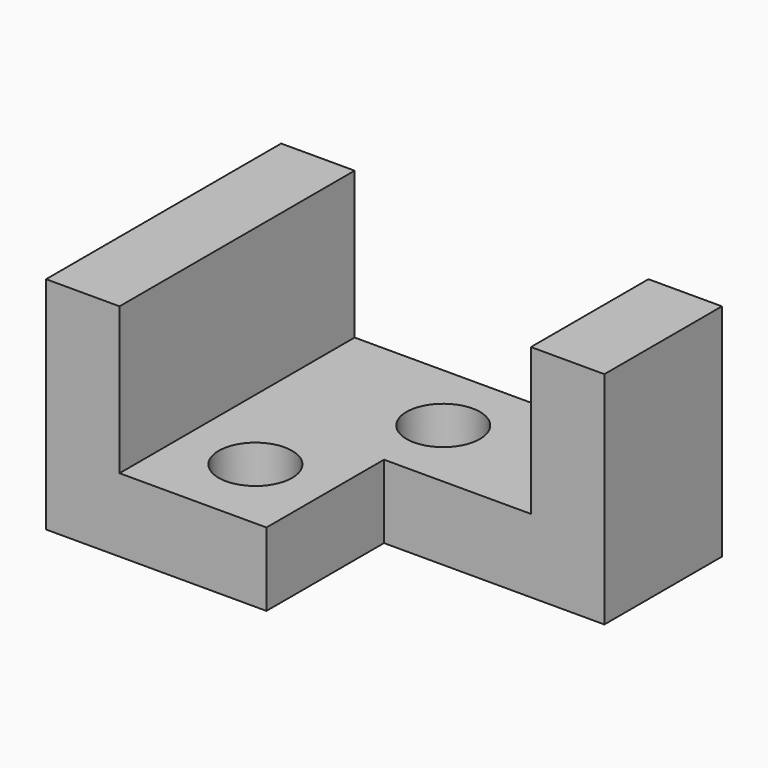
from build123d import *

# Parameters (mm, degrees)
F0_W      = 76.2
F0_H      = 12.7
F1_DEPTH  = 25.4
F3_DEPTH  = 50.8
F4_W      = 38.1
F4_H      = 12.7
F5_DEPTH  = 25.4
F6_W      = 12.7
F6_H      = 25.4
F7_DEPTH  = 25.4
F8_W      = 12.7
F8_H      = 50.8
F9_DEPTH  = 25.4
F10_R     = 6.35
F11_DEPTH = 25.4
F12_R     = 6.35
F13_DEPTH = 25.4


# Not quite as in the source:
# - a feature of the source that left no trace in its solid (it failed there, or was rolled back) is left out


with BuildPart() as f1:
    # F0 (on Front) → F1 (new body)
    with BuildSketch(Plane.XZ):
        with Locations((4.0105291711, 0)):
            Rectangle(F0_W, F0_H)
    extrude(amount=F1_DEPTH)

    # F0 (on Front) → F3 (join)
    with BuildSketch(Plane.XZ):
        with Locations((4.0105291711, 0)):
            Rectangle(F0_W, F0_H)
    extrude(amount=F3_DEPTH)

    # F4 (on face) → F5 (cut)
    with BuildSketch(Plane.XZ.offset(50.8)):
        with Locations((23.0605291711, 0)):
            Rectangle(F4_W, F4_H)
    extrude(amount=-F5_DEPTH, mode=Mode.SUBTRACT)

    # F6 (on face) → F7 (join)
    with BuildSketch(Plane.XY.offset(6.35)):
        with Locations((35.7605291711, -12.7)):
            Rectangle(F6_W, F6_H)
    extrude(amount=F7_DEPTH)

    # F8 (on face) → F9 (join)
    with BuildSketch(Plane.XY.offset(6.35)):
        with Locations((-27.7394708289, -25.4)):
            Rectangle(F8_W, F8_H)
    extrude(amount=F9_DEPTH)

    # F10 (on face) → F11 (cut)
    with BuildSketch(Plane.XY.offset(6.35)):
        with Locations((-8.6894708289, -37.3077057302)):
            Circle(F10_R)
    extrude(amount=-F11_DEPTH, mode=Mode.SUBTRACT)

    # F12 (on face) → F13 (cut)
    with BuildSketch(Plane.XY.offset(6.35)):
        with Locations((4.0105291711, -12.5951375812)):
            Circle(F12_R)
    extrude(amount=-F13_DEPTH, mode=Mode.SUBTRACT)


solid = f1.part
